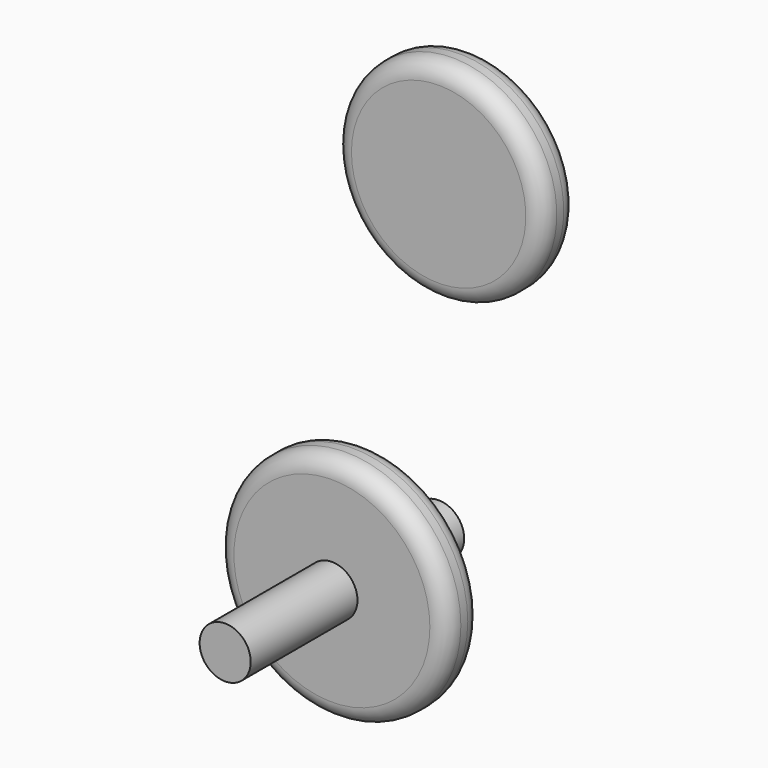
from build123d import *

# Parameters (mm, degrees)
F0_R     = 33.9914907239
F1_DEPTH = 12.7
F2_R     = 5.08
F3_R     = 7.5374575826
F4_DEPTH = 39.37
F7_R     = 30.8069471107
F8_DEPTH = 12.7
F9_R     = 5.08


# Not quite as in the source:
# - a feature of the source that left no trace in its solid (it failed there, or was rolled back) is left out


with BuildPart() as f1:
    # F0 (on Front) → F1 (new body)
    with BuildSketch(Plane.XZ):
        Circle(F0_R)
    extrude(amount=F1_DEPTH)

    # F2
    f2_edges = [f1.edges().sort_by_distance(p)[0] for p in [
        (-33.991491, -12.7, 0),
        (-33.991491, 0, 0),
    ]]
    fillet(f2_edges, radius=F2_R)

    # F3 (on face) → F4 (join, symmetric)
    with BuildSketch(Plane.XZ.offset(12.7)):
        Circle(F3_R)
    extrude(amount=F4_DEPTH, both=True)


with BuildPart() as f8:
    # F7 (on face) → F8 (new body)
    with BuildSketch(Plane(origin=(0, 26.67, 0), x_dir=(-1, 0, 0), z_dir=(0, 1, 0))):
        with Locations((0, 89.6297171712)):
            Circle(F7_R)
    extrude(amount=F8_DEPTH)

    # F9
    f9_edges = [f8.edges().sort_by_distance(p)[0] for p in [
        (30.806947, 39.37, 89.629717),
        (30.806947, 26.67, 89.629717),
    ]]
    fillet(f9_edges, radius=F9_R)


solid = Compound([f1.part, f8.part])
